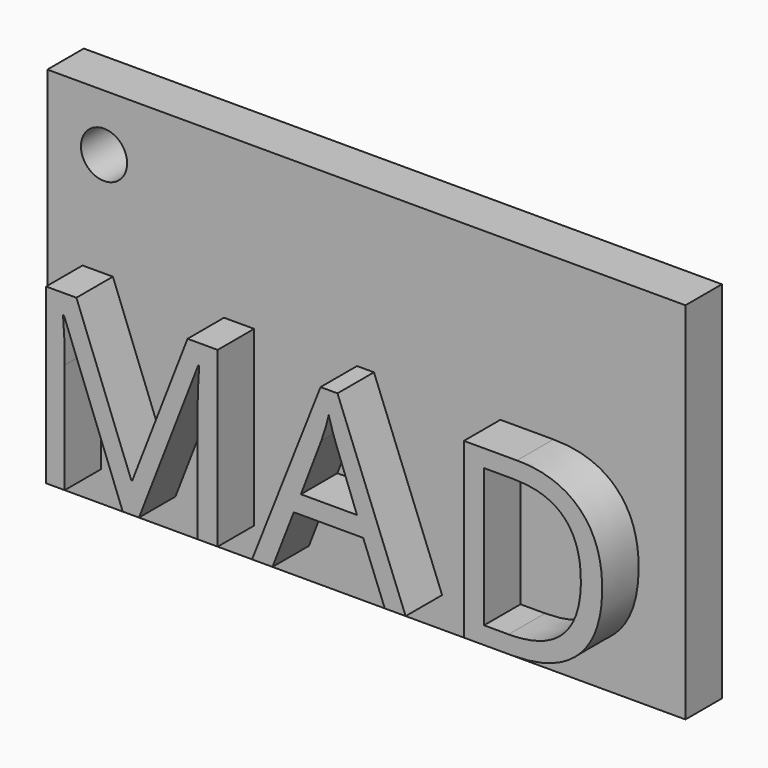
from build123d import *

# Parameters (mm, degrees)
F0_W         = 88.9
F0_H         = 50.8
F0_R         = 3.217766284
F1_DEPTH     = 6.35
F0_TEXT_SIZE = 33.8078720691
F2_DEPTH     = 12.7


# Not quite as in the source:
# - Text() gives the source's letters only with a copy of the font that has no kerning and outlines rounded to 1/6400 em; it was checked with that copy


with BuildPart() as f1:
    # F0 (on Front) → F1 (new body)
    with BuildSketch(Plane.XZ):
        with Locations((-1.5829317272, 8.5292911287)):
            Rectangle(F0_W, F0_H)
        with BuildLine():
            Line((-28.1859603332, -12.6373765164), (-30.4468617778, -12.6373765164))
            Line((-30.4468617778, -12.6373765164), (-38.6347057946, 8.7566675273))
            Line((-38.6347057946, 8.7566675273), (-38.7667677948, 8.7566675273))
            add(Edge.make_bspline(
                [(-38.7667677948, 8.7566675273), (-38.5343386744, 6.2157946421), (-38.5343386744, 2.7135103949)],
                knots=[0, 0, 0, 1, 1, 1], degree=2))
            Line((-38.5343386744, 2.7135103949), (-38.5343386744, -12.6373765164))
            Line((-38.5343386744, -12.6373765164), (-41.1280363597, -12.6373765164))
            Line((-41.1280363597, -12.6373765164), (-41.1280363597, 11.4982746529))
            Line((-41.1280363597, 11.4982746529), (-36.902052351, 11.4982746529))
            Line((-36.902052351, 11.4982746529), (-29.2583037754, -8.4113925078))
            Line((-29.2583037754, -8.4113925078), (-29.1262417751, -8.4113925078))
            Line((-29.1262417751, -8.4113925078), (-21.4191034394, 11.4982746529))
            Line((-21.4191034394, 11.4982746529), (-17.2248143108, 11.4982746529))
            Line((-17.2248143108, 11.4982746529), (-17.2248143108, -12.6373765164))
            Line((-17.2248143108, -12.6373765164), (-20.0298111965, -12.6373765164))
            Line((-20.0298111965, -12.6373765164), (-20.0298111965, 2.9142446354))
            add(Edge.make_bspline(
                [(-20.0298111965, 2.9142446354), (-20.0298111965, 5.5871795208), (-19.7973820761, 8.7249726472)],
                knots=[0, 0, 0, 1, 1, 1], degree=2))
            Line((-19.7973820761, 8.7249726472), (-19.9294440763, 8.7249726472))
            Line((-19.9294440763, 8.7249726472), (-28.1859603332, -12.6373765164))
        make_face(mode=Mode.SUBTRACT)
        Polygon((8.9631964449, -12.6373765164), (6.057832439, -12.6373765164), (3.0521013128, -4.9619330607), (-6.6201195869, -4.9619330607), (-9.588873353, -12.6373765164), (-12.4308475988, -12.6373765164), (-2.8906886993, 11.5986417731), (-0.5294201345, 11.5986417731), align=None, mode=Mode.SUBTRACT)
        with BuildLine():
            add(Edge.make_bspline(
                [(33.226200796, 8.3789702065), (36.3455052424, 5.2596657602), (36.3455052424, -0.3397630513)],
                knots=[0, 0, 0, 1, 1, 1], degree=2))
            add(Edge.make_bspline(
                [(36.3455052424, -0.3397630513), (36.3455052424, -6.3142479435), (33.1020625157, -9.47581223)],
                knots=[0, 0, 0, 1, 1, 1], degree=2))
            add(Edge.make_bspline(
                [(33.1020625157, -9.47581223), (29.8586197891, -12.6373765164), (23.7679203367, -12.6373765164)],
                knots=[0, 0, 0, 1, 1, 1], degree=2))
            Line((23.7679203367, -12.6373765164), (17.080300643, -12.6373765164))
            Line((17.080300643, -12.6373765164), (17.080300643, 11.4982746529))
            Line((17.080300643, 11.4982746529), (24.4757726581, 11.4982746529))
            add(Edge.make_bspline(
                [(24.4757726581, 11.4982746529), (30.1068963496, 11.4982746529), (33.226200796, 8.3789702065)],
                knots=[0, 0, 0, 1, 1, 1], degree=2))
        make_face(mode=Mode.SUBTRACT)
        with Locations((-38.1342619658, 26.0464213789)):
            Circle(F0_R, mode=Mode.SUBTRACT)
    extrude(amount=F1_DEPTH)



with BuildPart() as f1b:
    # F0 (on Front) → F1, piece 2 (new body)
    with BuildSketch(Plane.XZ):
        with BuildLine():
            add(Edge.make_bspline(
                [(30.8490847911, -7.7431587864), (33.3767514763, -5.2735993814), (33.3767514763, -0.4401301715)],
                knots=[0, 0, 0, 1, 1, 1], degree=2))
            add(Edge.make_bspline(
                [(33.3767514763, -0.4401301715), (33.3767514763, 4.2824069582), (31.0075591915, 6.6753704031)],
                knots=[0, 0, 0, 1, 1, 1], degree=2))
            add(Edge.make_bspline(
                [(31.0075591915, 6.6753704031), (28.6383669066, 9.0683338479), (23.9633720971, 9.0683338479)],
                knots=[0, 0, 0, 1, 1, 1], degree=2))
            Line((23.9633720971, 9.0683338479), (19.8852975287, 9.0683338479))
            Line((19.8852975287, 9.0683338479), (19.8852975287, -10.2127181915))
            Line((19.8852975287, -10.2127181915), (23.3030620957, -10.2127181915))
            add(Edge.make_bspline(
                [(23.3030620957, -10.2127181915), (28.321418106, -10.2127181915), (30.8490847911, -7.7431587864)],
                knots=[0, 0, 0, 1, 1, 1], degree=2))
        make_face()
    extrude(amount=F1_DEPTH)


with BuildPart() as f1c:
    # F0 (on Front) → F1, piece 3 (new body)
    with BuildSketch(Plane.XZ):
        with BuildLine():
            Line((-5.6270133449, -2.4369076156), (2.1804921111, -2.4369076156))
            Line((2.1804921111, -2.4369076156), (-0.6297872547, 5.0430840797))
            add(Edge.make_bspline(
                [(-0.6297872547, 5.0430840797), (-1.1738826958, 6.4640712026), (-1.749673017, 8.5242384068)],
                knots=[0, 0, 0, 1, 1, 1], degree=2))
            add(Edge.make_bspline(
                [(-1.749673017, 8.5242384068), (-2.1141641377, 6.9394944036), (-2.7903215791, 5.0430840797)],
                knots=[0, 0, 0, 1, 1, 1], degree=2))
            Line((-2.7903215791, 5.0430840797), (-5.6270133449, -2.4369076156))
        make_face()
    extrude(amount=F1_DEPTH)


with BuildPart() as f1_1:
    add(f1.part)

    add(f1b.part)  # F2 merges F1b

    add(f1c.part)  # F2 merges F1c
    # F0 (on Front) → F2 (join)
    with BuildSketch(Plane.XZ):
        with Locations((13.7629031962, -12.6373765164)):
            Text('D', F0_TEXT_SIZE, font='Open Sans', text_align=(TextAlign.LEFT, TextAlign.BOTTOM))
        with Locations((-12.4308475988, -12.6373765164)):
            Text('A', F0_TEXT_SIZE, font='Open Sans', text_align=(TextAlign.LEFT, TextAlign.BOTTOM))
        with Locations((-44.4454338065, -12.6373765164)):
            Text('M', F0_TEXT_SIZE, font='Open Sans', text_align=(TextAlign.LEFT, TextAlign.BOTTOM))
    extrude(amount=F2_DEPTH)


solid = f1_1.part
